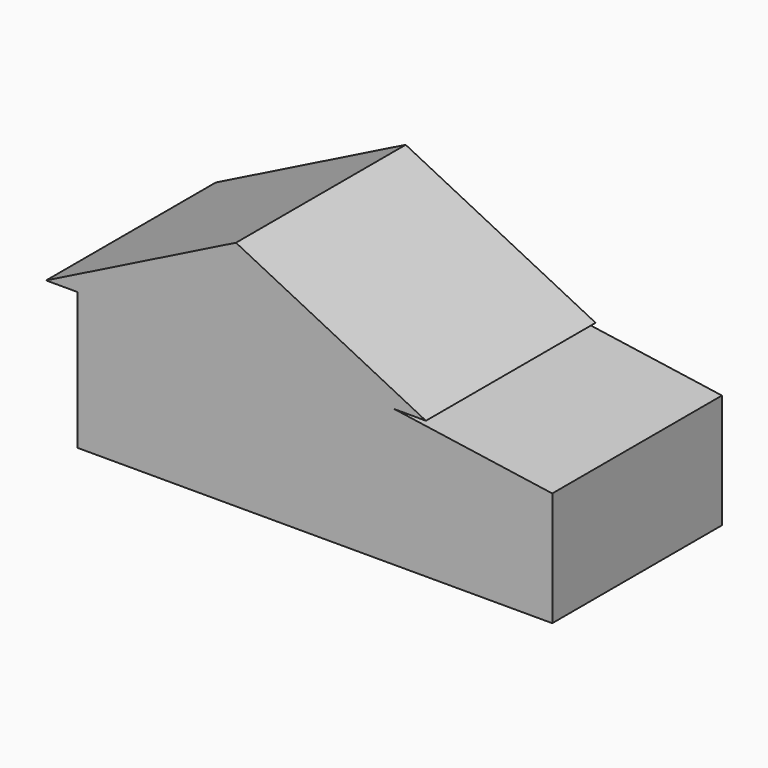
from build123d import *

# Parameters (mm, degrees)
F0_W          = 2743.2
F0_H          = 1371.6
F0_W_2        = 1219.2
F0_H_2        = 761.5693855479
F0_W_3        = 4563.8048175471
F0_H_3        = 609.6
F0_W_4        = 914.4
F0_H_4        = 2133.6
F1_DEPTH      = 6096
F1_DEPTH_BACK = 30.48


# Not quite as in the source:
# - the program builds the solid bodies; features that only make, move or delete a surface that nothing else refers to are left out


with BuildPart() as f1:
    # F0 (on Front) → F1 (new body, two sides)
    with BuildSketch(Plane.XZ) as f1_sk:
        Polygon((4572, 0), (0, 0), (-4572, 0), (-4572, -3352.8), (-3352.8, -3352.8), (-3352.8, -1219.2), (-2438.4, -1219.2), (-2438.4, -3352.8), (4572, -3352.8), (4572, -401.1528193951), align=None)
        with Locations((1981.2, -1359.7689430237)):
            Rectangle(F0_W, F0_H, mode=Mode.SUBTRACT)
        Polygon((9135.8048175471, -1063.5435686586), (4572, -401.1528193951), (4572, -3352.8), (9135.8048175471, -3352.8), align=None)
        with Locations((6349.5722342422, -2210.4459216781)):
            Rectangle(F0_W_2, F0_H_2, mode=Mode.SUBTRACT)
        Polygon((-3352.8, -3352.8), (-4572, -3352.8), (-4572, -3962.4), (4572, -3962.4), (4572, -3352.8), (-2438.4, -3352.8), align=None)
        Polygon((-4572, 0), (0, 0), (0, 2286), align=None)
        Polygon((0, 2286), (0, 0), (4572, 0), align=None)
        with Locations((1981.2, -1359.7689430237)):
            Rectangle(F0_W, F0_H)
        with Locations((6853.9024087735, -3657.6)):
            Rectangle(F0_W_3, F0_H_3)
        Polygon((-5486.4, 0), (-4572, 0), (0, 2286), (0, 2743.2), align=None)
        Polygon((0, 2286), (4572, 0), (5486.4, 0), (0, 2743.2), align=None)
        with Locations((-2895.6, -2286)):
            Rectangle(F0_W_4, F0_H_4)
        Polygon((9135.8048175471, -662.3907492636), (4572, 0), (4572, -401.1528193951), (9135.8048175471, -1063.5435686586), align=None)
        with Locations((6349.5722342422, -2210.4459216781)):
            Rectangle(F0_W_2, F0_H_2)
    extrude(amount=F1_DEPTH)
    extrude(f1_sk.sketch, amount=-F1_DEPTH_BACK)


solid = f1.part
